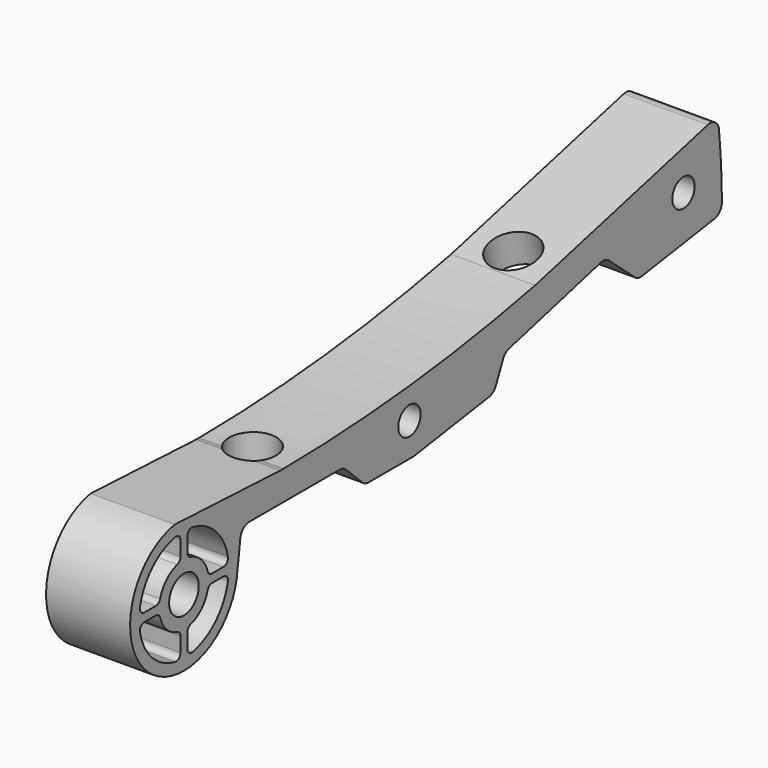
from build123d import *

# Parameters (mm, degrees)
F0_R     = 3.3
F0_R_2   = 2.5
F1_DEPTH = 15
F2_R     = 4.25
F3_DEPTH = 7.6
F4_R     = 4.25
F5_DEPTH = 15.8


# Not quite as in the source:
# - a feature names something its author has since deleted; it is built from what else it names


with BuildPart() as f1:
    # F0 (on Right) → F1 (new body)
    with BuildSketch(Plane.YZ):
        with BuildLine():
            ThreePointArc((21.8315579223, 10.717182122), (21.897134346, 10.7177196915), (21.9626931438, 10.7193322557))
            ThreePointArc((21.9626931438, 10.7193322557), (21.9630378123, 10.7252568669), (21.9633808826, 10.731181571))
            ThreePointArc((21.9633808826, 10.731181571), (21.7716697335, 10.7299327404), (21.5799577929, 10.728811993))
            Line((21.5799577929, 10.728811993), (21.8315579223, 10.717182122))
        make_face()
        with BuildLine():
            ThreePointArc((22.1844688263, 10.7327808001), (22.0736743793, 10.7245163933), (21.9626931438, 10.7193322557))
            ThreePointArc((21.9626931438, 10.7193322557), (21.897134346, 10.7177196915), (21.8315579223, 10.717182122))
            ThreePointArc((21.8315579223, 10.717182122), (21.6468606164, 10.7214485341), (21.4625573078, 10.7342386694))
            Line((21.4625573078, 10.7342386694), (-2.0614712889, 11.8216046341))
            ThreePointArc((-2.0614712889, 11.8216046341), (-7.9885695505, -8.9544824829), (11.9792964571, -0.7045966171))
            ThreePointArc((11.9792964571, -0.7045966171), (12.0074816864, -0.4822378377), (12.0652655082, -0.2656763826))
            Line((12.0652655082, -0.2656763826), (12.5823545671, 3.7402298466))
            ThreePointArc((12.5823545671, 3.7402298466), (13.2453067327, 4.9862024463), (14.565897859, 5.4841907695))
            Line((14.565897859, 5.4841907695), (34.746018001, 5.4841907695))
            ThreePointArc((34.746018001, 5.4841907695), (35.4911723527, 5.3401931919), (36.1290262829, 4.9289357615))
            Line((36.1290262829, 4.9289357615), (39.7961525429, 1.4185128035))
            ThreePointArc((39.7961525429, 1.4185128035), (40.4340064731, 1.0072553731), (41.1791608249, 0.8632577956))
            Line((41.1791608249, 0.8632577956), (51.1560065331, 0.8632577956))
            ThreePointArc((51.1560065331, 0.8632577956), (51.3046360431, 0.8687881245), (51.452443583, 0.8853485268))
            Line((51.452443583, 0.8853485268), (68.043755982, 3.3719538424))
            ThreePointArc((68.043755982, 3.3719538424), (68.9480745213, 3.750430082), (69.5639006382, 4.5131846154))
            Line((69.5639006382, 4.5131846154), (71.1927053136, 8.0496168184))
            ThreePointArc((71.1927053136, 8.0496168184), (71.7304115705, 8.7506241115), (72.5176709464, 9.151575379))
            Line((72.5176709464, 9.151575379), (93.0016589096, 14.3460792675))
            ThreePointArc((93.0016589096, 14.3460792675), (93.9531599103, 14.3538506609), (94.800564285, 13.9210454222))
            Line((94.800564285, 13.9210454222), (100.5567479715, 8.9494668086))
            ThreePointArc((100.5567479715, 8.9494668086), (101.3078443235, 8.5419637232), (102.1604743235, 8.4851607509))
            Line((102.1604743235, 8.4851607509), (118.2931486533, 10.9030281733))
            ThreePointArc((118.2931486533, 10.9030281733), (119.516973098, 11.5813971433), (119.9966558679, 12.8958685851))
            ThreePointArc((119.9966558679, 12.8958685851), (119.8113324935, 18.7264110882), (119.3428752162, 24.5410579746))
            ThreePointArc((119.3428752162, 24.5410579746), (118.5020303548, 25.9696085801), (116.872434029, 26.2732411356))
            Line((116.872434029, 26.2732411356), (78.344444671, 16.7187866332))
            ThreePointArc((78.344444671, 16.7187866332), (50.4120849121, 12.3407543123), (22.1844688263, 10.7327808001))
        make_face()
        with BuildLine():
            ThreePointArc((-9.8092514957, -1.9438583008), (-9.6011089256, -1.114801623), (-8.8283263462, -0.7494724707))
            Line((-8.8283263462, -0.7494724707), (-6.2601394612, -0.7494724707))
            ThreePointArc((-6.2601394612, -0.7494724707), (-5.6556353715, -0.9528704337), (-5.2970410826, -1.4803228598))
            ThreePointArc((-5.2970410826, -1.4803228598), (-3.8892204731, -3.8889541154), (-1.4806856428, -5.2969396851))
            ThreePointArc((-1.4806856428, -5.2969396851), (-0.9532704937, -5.6555533383), (-0.7499012145, -6.2600460414))
            Line((-0.7499012145, -6.2600460414), (-0.7499690502, -8.8282543402))
            ThreePointArc((-0.7499690502, -8.8282543402), (-1.1153301427, -9.6010367371), (-1.9444100554, -9.8091421407))
            ThreePointArc((-1.9444100554, -9.8091421407), (-7.0712666783, -7.0708689399), (-9.8092514957, -1.9438583008))
        make_face(mode=Mode.SUBTRACT)
        with BuildLine():
            ThreePointArc((9.8092514957, -1.9438583008), (7.0710678119, -7.0710678119), (1.9438583008, -9.8092514957))
            ThreePointArc((1.9438583008, -9.8092514957), (1.114801623, -9.6011089256), (0.7494724707, -8.8283263462))
            Line((0.7494724707, -8.8283263462), (0.7494724707, -6.2601394612))
            ThreePointArc((0.7494724707, -6.2601394612), (0.9528704337, -5.6556353715), (1.4803228598, -5.2970410826))
            ThreePointArc((1.4803228598, -5.2970410826), (3.8890872965, -3.8890872965), (5.2970410826, -1.4803228598))
            ThreePointArc((5.2970410826, -1.4803228598), (5.6556353715, -0.9528704337), (6.2601394612, -0.7494724707))
            Line((6.2601394612, -0.7494724707), (8.8283263462, -0.7494724707))
            ThreePointArc((8.8283263462, -0.7494724707), (9.6011089256, -1.114801623), (9.8092514957, -1.9438583008))
        make_face(mode=Mode.SUBTRACT)
        Circle(F0_R, mode=Mode.SUBTRACT)
        with BuildLine():
            Line((-6.2601394612, 0.7494724707), (-8.8283263462, 0.7494724707))
            ThreePointArc((-8.8283263462, 0.7494724707), (-9.6011089256, 1.114801623), (-9.8092514957, 1.9438583008))
            ThreePointArc((-9.8092514957, 1.9438583008), (-7.0710799085, 7.0710557152), (-1.9438918628, 9.8092448448))
            ThreePointArc((-1.9438918628, 9.8092448448), (-1.1148229448, 9.6010956435), (-0.7495026768, 8.8282939467))
            Line((-0.7495026768, 8.8282939467), (-0.7495705125, 6.2600856479))
            ThreePointArc((-0.7495705125, 6.2600856479), (-0.9529717251, 5.6556036891), (-1.480405818, 5.2970178982))
            ThreePointArc((-1.480405818, 5.2970178982), (-3.8891177504, 3.8890568424), (-5.2970410826, 1.4803228598))
            ThreePointArc((-5.2970410826, 1.4803228598), (-5.6556353715, 0.9528704337), (-6.2601394612, 0.7494724707))
        make_face(mode=Mode.SUBTRACT)
        with BuildLine():
            Line((0.7494724707, 6.2601394612), (0.7494724707, 8.8283263462))
            ThreePointArc((0.7494724707, 8.8283263462), (1.114801623, 9.6011089256), (1.9438583008, 9.8092514957))
            ThreePointArc((1.9438583008, 9.8092514957), (7.0710678119, 7.0710678119), (9.8092514957, 1.9438583008))
            ThreePointArc((9.8092514957, 1.9438583008), (9.6011089256, 1.114801623), (8.8283263462, 0.7494724707))
            Line((8.8283263462, 0.7494724707), (6.2601394612, 0.7494724707))
            ThreePointArc((6.2601394612, 0.7494724707), (5.6556353715, 0.9528704337), (5.2970410826, 1.4803228598))
            ThreePointArc((5.2970410826, 1.4803228598), (3.8890872965, 3.8890872965), (1.4803228598, 5.2970410826))
            ThreePointArc((1.4803228598, 5.2970410826), (0.9528704337, 5.6556353715), (0.7494724707, 6.2601394612))
        make_face(mode=Mode.SUBTRACT)
        with Locations((50.3031872213, 6.8563437089)):
            Circle(F0_R_2, mode=Mode.SUBTRACT)
        with Locations((111.4225909114, 17.8264938295)):
            Circle(F0_R_2, mode=Mode.SUBTRACT)
        with BuildLine():
            ThreePointArc((21.9633808826, 10.731181571), (21.9630378123, 10.7252568669), (21.9626931438, 10.7193322557))
            ThreePointArc((21.9626931438, 10.7193322557), (22.0736743793, 10.7245163933), (22.1844688263, 10.7327808001))
            ThreePointArc((22.1844688263, 10.7327808001), (22.0739250085, 10.7319598925), (21.9633808826, 10.731181571))
        make_face()
        with BuildLine():
            ThreePointArc((21.4625573078, 10.7342386694), (21.6468606164, 10.7214485341), (21.8315579223, 10.717182122))
            Line((21.8315579223, 10.717182122), (21.5799577929, 10.728811993))
            Line((21.5799577929, 10.728811993), (21.4625573078, 10.7342386694))
        make_face()
    extrude(amount=F1_DEPTH)

    # F2 (on face) → F3 (cut)
    with BuildSketch(Plane(origin=(0, 0, 5.4841907695), x_dir=(1, 0, 0), z_dir=(0, 0, -1))):
        with Locations((7.5, -24.65595793)):
            Circle(F2_R)
    extrude(amount=-F3_DEPTH, mode=Mode.SUBTRACT)

    # F4 (on face) → F5 (cut)
    with BuildSketch(Plane(origin=(0, 2.2011211845, -8.6798933673), x_dir=(1, 0, 0), z_dir=(0, 0.2458080366, -0.9693185282))):
        with Locations((7.5, -84.6746127131)):
            Circle(F4_R)
    extrude(amount=-F5_DEPTH, mode=Mode.SUBTRACT)


solid = f1.part
